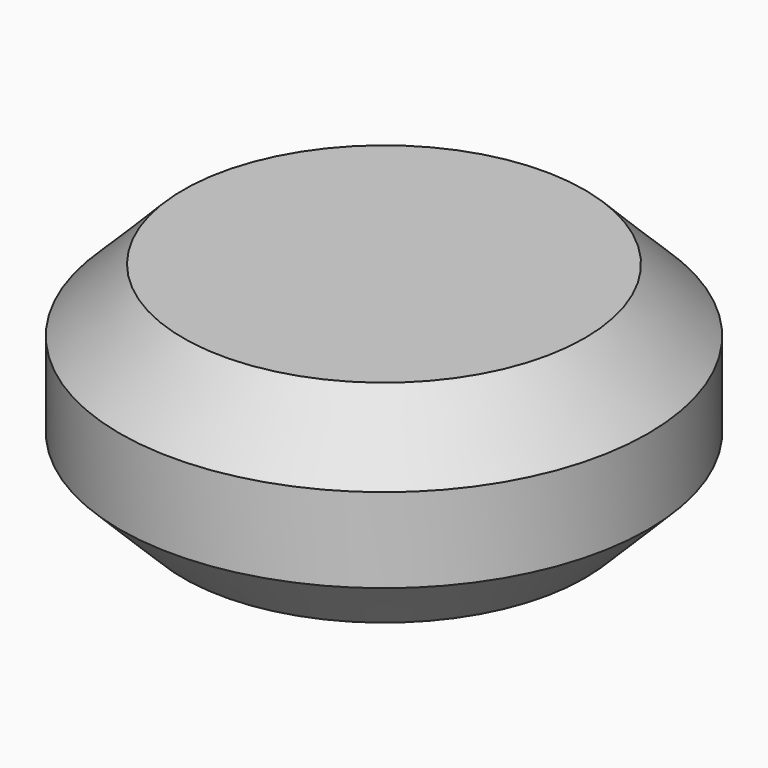
from build123d import *

# Parameters (mm, degrees)
F0_R     = 12.5
F1_DEPTH = 10
F2_SIZE  = 3
F3_R     = 5.25
F4_DEPTH = 8


# Not quite as in the source:
# - a feature names something its author has since deleted; it is built from what else it names


with BuildPart() as f1:
    # F0 (on Top) → F1 (new body)
    with BuildSketch(Plane.XY):
        Circle(F0_R)
    extrude(amount=F1_DEPTH)

    # F2
    f2_edges = [f1.edges().sort_by_distance(p)[0] for p in [
        (-12.5, 0, 10),
        (12.5, 0, 5),
        (-12.5, 0, 0),
    ]]
    chamfer(f2_edges, length=F2_SIZE)

    # F3 (on face) → F4 (cut)
    with BuildSketch(Plane(origin=(0, 0, 0), x_dir=(1, 0, 0), z_dir=(0, 0, -1))):
        Circle(F3_R)
    extrude(amount=-F4_DEPTH, mode=Mode.SUBTRACT)


solid = f1.part
